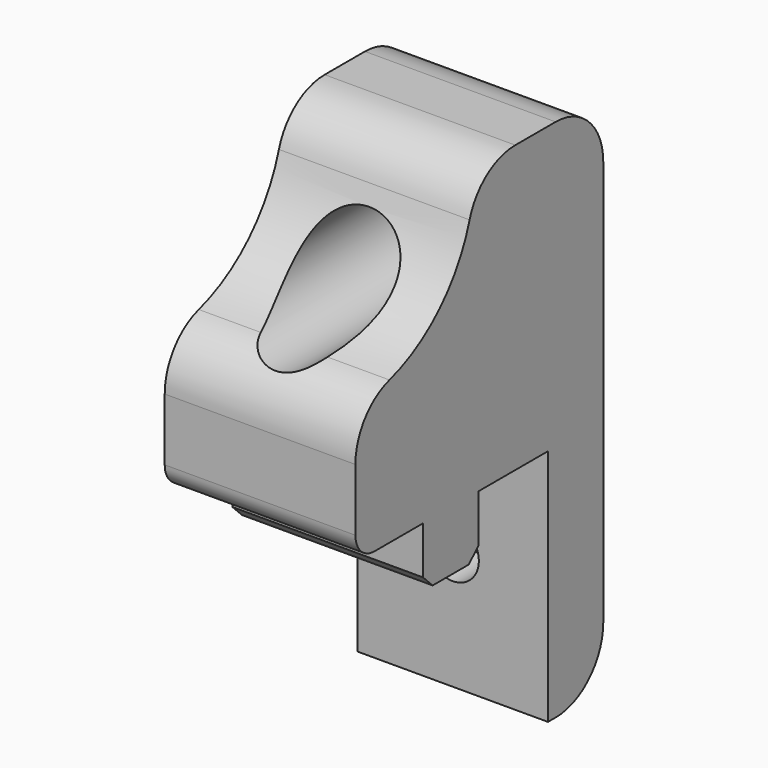
from build123d import *

# Parameters (mm, degrees)
F0_W           = 16
F0_H           = 24
F1_DEPTH       = 13
F2_W           = 16
F2_H           = 5.8
F3_DEPTH       = 5
F4_DEPTH       = 20
F5_R           = 4.05
F6_DEPTH       = 20
F8_D           = 4.4
F8_CBORE_D     = 8.25
F8_CBORE_DEPTH = 2
F9_SIZE        = 1
F11_DEPTH      = 16.001
F12_T1_DEPTH   = 27.2312288127
F12_T3_DEPTH   = 27.2312288127
F12_T5_DEPTH   = 41
F12_T7_DEPTH   = 37.3525491562
F13_R          = 2


# Not quite as in the source:
# - a fillet or chamfer that OpenCascade refuses, or shapes differently, is made with other operations: its cross-section is extruded or revolved along the edge and cut away or added
# - a feature names something its author has since deleted; it is built from what else it names


with BuildPart() as f1:
    # F0 (on Front) → F1 (new body, symmetric)
    with BuildSketch(Plane.XZ):
        Rectangle(F0_W, F0_H)
    extrude(amount=F1_DEPTH, both=True)

    # F2 (on face) → F3 (join)
    with BuildSketch(Plane(origin=(0, 0, -12), x_dir=(1, 0, 0), z_dir=(0, 0, -1))):
        with Locations((0, 3)):
            Rectangle(F2_W, F2_H)
    extrude(amount=F3_DEPTH)

    # F2 (on face) → F4 (join)
    with BuildSketch(Plane(origin=(0, 0, -12), x_dir=(1, 0, 0), z_dir=(0, 0, -1))):
        with Locations((0, -10.1)):
            Rectangle(F2_W, F2_H)
    extrude(amount=F4_DEPTH)

    # F5 (on face) → F6 (cut)
    with BuildSketch(Plane.XZ.offset(13)):
        with Locations((0, 2.95)):
            Circle(F5_R)
    extrude(amount=-F6_DEPTH, mode=Mode.SUBTRACT)

    # F8 (through all)
    with Locations(Plane(origin=(0, 13, 0), x_dir=(-1, 0, 0), z_dir=(0, 1, 0))):
        with Locations((0, -22)):
            CounterBoreHole(F8_D / 2, F8_CBORE_D / 2, F8_CBORE_DEPTH)

    # F9
    f9_edges = [f1.edges().sort_by_distance(p)[0] for p in [
        (0, -5.9, -17),
        (0, -0.1, -17),
    ]]
    chamfer(f9_edges, length=F9_SIZE)

    # F10 (on face) → F11 (cut, through all)
    with BuildSketch(Plane.YZ.offset(8)):
        with BuildLine():
            Line((-13, 12), (-0.5, 12))
            ThreePointArc((-0.5, 12), (-21.8388347648, 20.8388347648), (-13, -0.5))
            Line((-13, -0.5), (-13, 12))
        make_face()
        with BuildLine():
            ThreePointArc((-13, -0.5), (-4.1611652352, 3.1611652352), (-0.5, 12))
            Line((-0.5, 12), (-13, 12))
            Line((-13, 12), (-13, -0.5))
        make_face()
    extrude(amount=-F11_DEPTH, mode=Mode.SUBTRACT)

    # F12: fillet of radius 5 on 5 edges, made by hand

    # F12_s2 → F12_t1 (cut)
    with BuildSketch(Plane.YZ.offset(-8.5549542346)):
        with BuildLine():
            ThreePointArc((-9.4285714286, 0.0210644063), (-12.0089186287, -1.7824383079), (-13, -4.7705098312))
            Line((-13, -4.7705098312), (-13, -0.5))
            ThreePointArc((-13, -0.5), (-11.1953802231, -0.369047961), (-9.4285714286, 0.0210644063))
        make_face()
    extrude(amount=F12_T1_DEPTH, mode=Mode.SUBTRACT)

    # F12_s4 → F12_t3 (cut)
    with BuildSketch(Plane.YZ.offset(-18.6762745781)):
        with BuildLine():
            ThreePointArc((-9.4285714286, 0.0210644063), (-12.0089186287, -1.7824383079), (-13, -4.7705098312))
            Line((-13, -4.7705098312), (-13, -0.5))
            ThreePointArc((-13, -0.5), (-11.1953802231, -0.369047961), (-9.4285714286, 0.0210644063))
        make_face()
    extrude(amount=F12_T3_DEPTH, mode=Mode.SUBTRACT)

    # F12_s6 → F12_t5 (cut)
    with BuildSketch(Plane.YZ.offset(-20.5)):
        with BuildLine():
            ThreePointArc((8, -32), (11.5355339059, -30.5355339059), (13, -27))
            Line((13, -27), (13, -32))
            Line((13, -32), (8, -32))
        make_face()
        with BuildLine():
            ThreePointArc((13, 7), (11.5355339059, 10.5355339059), (8, 12))
            Line((8, 12), (13, 12))
            Line((13, 12), (13, 7))
        make_face()
    extrude(amount=F12_T5_DEPTH, mode=Mode.SUBTRACT)

    # F12_s8 → F12_t7 (cut)
    with BuildSketch(Plane.YZ.offset(-18.6762745781)):
        with BuildLine():
            ThreePointArc((3.7705098312, 12), (0.7824383079, 11.0089186287), (-1.0210644063, 8.4285714286))
            ThreePointArc((-1.0210644063, 8.4285714286), (-0.630952039, 10.1953802231), (-0.5, 12))
            Line((-0.5, 12), (3.7705098312, 12))
        make_face()
    extrude(amount=F12_T7_DEPTH, mode=Mode.SUBTRACT)

    # F13
    f13_edges = [f1.edges().sort_by_distance(p)[0] for p in [
        (0, -13, -12),
    ]]
    fillet(f13_edges, radius=F13_R)


solid = f1.part
